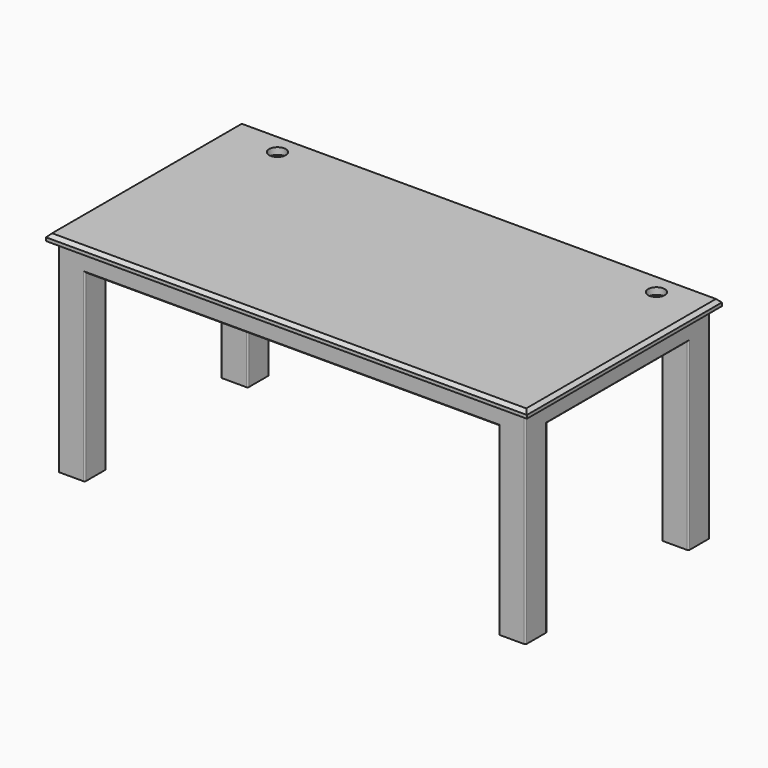
from build123d import *

# Parameters (mm, degrees)
F1_W        = 1828.8
F1_H        = 927.1
F2_DEPTH    = 25.4
F0_W        = 1778
F0_H        = 876.3
F3_DEPTH    = 101.6
F4_W        = 101.6
F4_H        = 101.6
F5_DEPTH    = 698.5
F6_T        = 25.4
F6_T3_DEPTH = 927.1
F6_T5_DEPTH = 1828.8
F7_R        = 31.75
F8_DEPTH    = 25.4
F9_SIZE     = 12.7
F10_R       = 5.08
F11_SIZE    = 5.08


# Not quite as in the source:
# - a shell that OpenCascade refuses in one call is made with other operations: the cavity is built on its own and cut out


with BuildPart() as f2:
    # F1 (on Top) → F2 (new body)
    with BuildSketch(Plane.XY):
        Rectangle(F1_W, F1_H)
    extrude(amount=-F2_DEPTH)

    # F0 (on Top) → F3 (join)
    with BuildSketch(Plane.XY):
        Rectangle(F0_W, F0_H)
    extrude(amount=-F3_DEPTH)

    # F4 (on face) → F5 (join)
    with BuildSketch(Plane(origin=(0, 0, -101.6), x_dir=(1, 0, 0), z_dir=(0, 0, -1))):
        with Locations((-838.2, 387.35)):
            Rectangle(F4_W, F4_H)
        with Locations((-838.2, -387.35)):
            Rectangle(F4_W, F4_H)
        with Locations((838.2, 387.35)):
            Rectangle(F4_W, F4_H)
        with Locations((838.2, -387.35)):
            Rectangle(F4_W, F4_H)
    extrude(amount=F5_DEPTH)

    # F6: shell of thickness 25.4, made by hand


with BuildPart() as f6_core1:
    # F6_t2: copy of F2
    add(f2.part)

    # the walls: a layer under each face that stays
    f6_faces = [f6_core1.faces().sort_by_distance(p)[0] for p in [
        (0, 463.55, -12.7),
        (628.65, -452.1043209877, -25.4),
        (762, 438.15, -80.7357142857),
        (-838.2, 387.35, -800.1),
        (-838.2, 336.55, -450.85),
        (-787.4, 387.35, -450.85),
        (-838.2, -336.55, -450.85),
        (-838.2, -387.35, -800.1),
        (-787.4, -387.35, -450.85),
        (787.4, -387.35, -450.85),
        (838.2, -387.35, -800.1),
        (838.2, -336.55, -450.85),
        (838.2, 336.55, -450.85),
        (787.4, 387.35, -450.85),
        (838.2, 387.35, -800.1),
        (889, -375.5571428571, -744.7642857143),
        (-762, -438.15, -80.7357142857),
        (-889, 375.5571428571, -744.7642857143),
        (0, -463.55, -12.7),
        (0, 0, 0),
        (-914.4, 0, -12.7),
        (914.4, 0, -12.7),
    ]]
    thicken(f6_faces, amount=-F6_T, mode=Mode.SUBTRACT)

    # F6_s4 → F6_t3 (cut)
    with BuildSketch(Plane.XZ.offset(-463.55)):
        Polygon((-889.254, -25.654), (-889, 0), (-863.6, 0), (-863.6, -25.4), align=None)
        Polygon((889.254, -25.654), (889, 0), (863.6, 0), (863.6, -25.4), align=None)
    extrude(amount=F6_T3_DEPTH, mode=Mode.SUBTRACT)

    # F6_s6 → F6_t5 (cut)
    with BuildSketch(Plane.YZ.offset(-914.4)):
        Polygon((-438.404, -25.654), (-438.15, 0), (-412.75, 0), (-412.75, -25.4), align=None)
        Polygon((438.404, -25.654), (438.15, 0), (412.75, 0), (412.75, -25.4), align=None)
    extrude(amount=F6_T5_DEPTH, mode=Mode.SUBTRACT)


with BuildPart() as f2_1:
    add(f2.part)

    # what is left inside the walls is the cavity
    f6_cavity = [f6_core1.part.solids().sort_by_distance(p)[0] for p in [
        (0, -137.583333, -25.654),
    ]]
    add(f6_cavity, mode=Mode.SUBTRACT)

    # F7 (on face) → F8 (cut)
    with BuildSketch(Plane.XY):
        with Locations((-704.85, 374.65)):
            Circle(F7_R)
        with Locations((736.6, 374.65)):
            Circle(F7_R)
    extrude(amount=-F8_DEPTH, mode=Mode.SUBTRACT)

    # F9
    f9_edges = [f2_1.edges().sort_by_distance(p)[0] for p in [
        (0, -463.55, 0),
        (-914.4, 0, 0),
        (0, 463.55, 0),
        (914.4, 0, 0),
    ]]
    chamfer(f9_edges, length=F9_SIZE)

    # F10
    f10_edges = [f2_1.edges().sort_by_distance(p)[0] for p in [
        (-889, -438.15, -412.75),
        (-787.4, -438.15, -450.85),
        (-889, -336.55, -450.85),
        (-787.4, -336.55, -450.85),
        (787.4, -438.15, -450.85),
        (889, -438.15, -412.75),
        (787.4, -336.55, -450.85),
        (889, -336.55, -450.85),
        (889, 336.55, -450.85),
        (787.4, 336.55, -450.85),
        (889, 438.15, -412.75),
        (787.4, 438.15, -450.85),
        (-889, 438.15, -412.75),
        (-787.4, 438.15, -450.85),
        (-889, 336.55, -450.85),
        (-787.4, 336.55, -450.85),
    ]]
    fillet(f10_edges, radius=F10_R)

    # F11
    f11_edges = [f2_1.edges().sort_by_distance(p)[0] for p in [
        (-889, 0, -101.6),
        (0, -438.15, -101.6),
        (889, 0, -101.6),
        (0, 438.15, -101.6),
    ]]
    chamfer(f11_edges, length=F11_SIZE)


solid = f2_1.part
